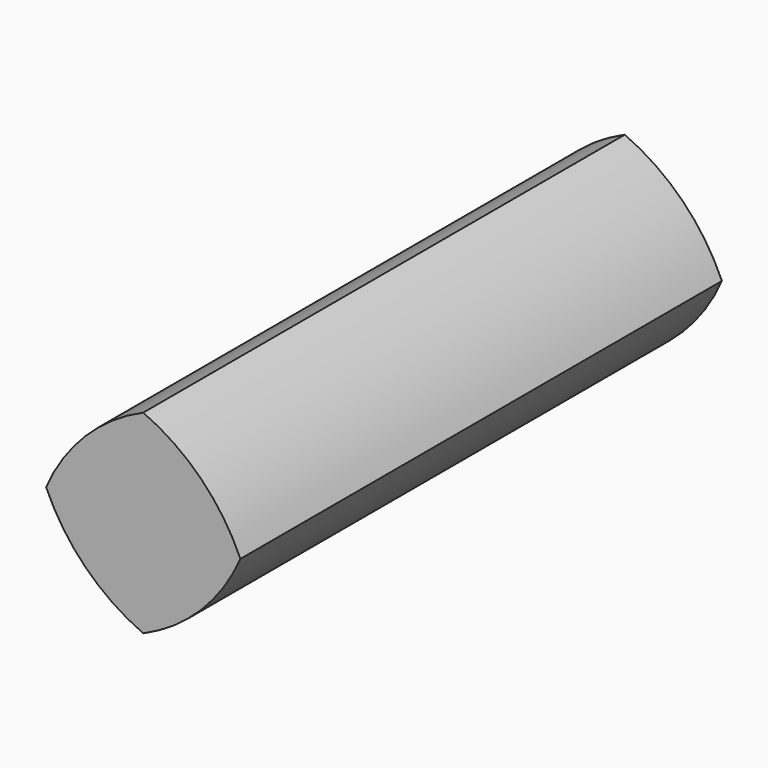
from build123d import *

# Parameters (mm, degrees)
F0_W        = 203.2
F0_H        = 76.2
F1_DEPTH    = 76.2
F2_T1_DEPTH = 520.7


# Not quite as in the source:
# - a fillet or chamfer that OpenCascade refuses, or shapes differently, is made with other operations: its cross-section is extruded or revolved along the edge and cut away or added


with BuildPart() as f1:
    # F0 (on Right) → F1 (new body)
    with BuildSketch(Plane.YZ):
        Rectangle(F0_W, F0_H)
    extrude(amount=F1_DEPTH)

    # F2: fillet of radius 63.5 on 4 edges, made by hand

    # F2_s2 → F2_t1 (cut)
    with BuildSketch(Plane.XZ.offset(-260.35)):
        with BuildLine():
            ThreePointArc((63.5, 38.1), (18.5987193947, 19.5012806053), (0, -25.4))
            Line((0, -25.4), (0, 38.1))
            Line((0, 38.1), (63.5, 38.1))
        make_face()
        with BuildLine():
            ThreePointArc((63.5, -38.1), (18.5987193947, -19.5012806053), (0, 25.4))
            Line((0, 25.4), (0, -38.1))
            Line((0, -38.1), (63.5, -38.1))
        make_face()
        with BuildLine():
            ThreePointArc((12.7, 38.1), (57.6012806053, 19.5012806053), (76.2, -25.4))
            Line((76.2, -25.4), (76.2, 38.1))
            Line((76.2, 38.1), (12.7, 38.1))
        make_face()
        with BuildLine():
            ThreePointArc((12.7, -38.1), (57.6012806053, -19.5012806053), (76.2, 25.4))
            Line((76.2, 25.4), (76.2, -38.1))
            Line((76.2, -38.1), (12.7, -38.1))
        make_face()
    extrude(amount=F2_T1_DEPTH, mode=Mode.SUBTRACT)


solid = f1.part
